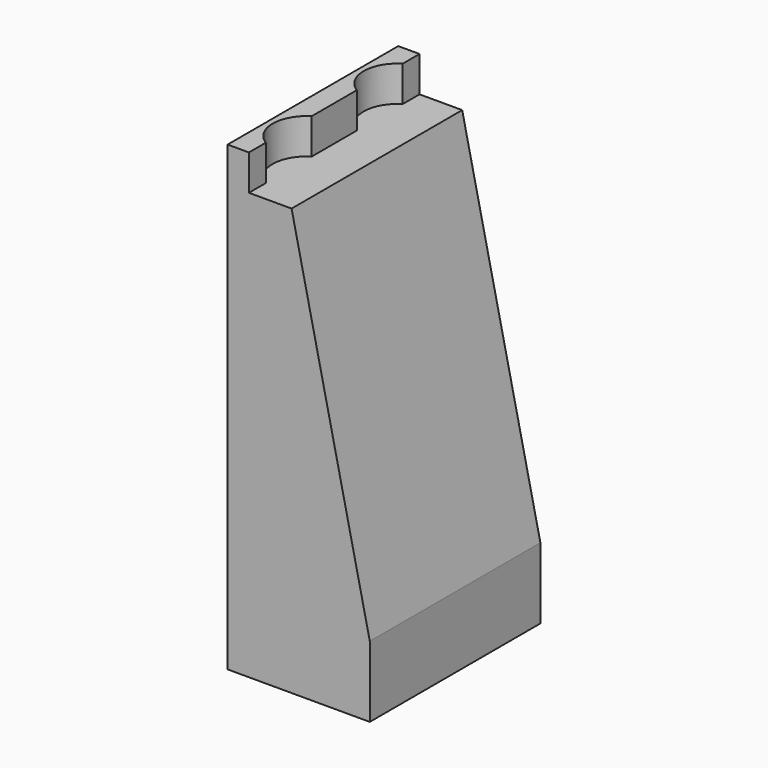
from build123d import *

# Parameters (mm, degrees)
F0_W      = 20
F0_H      = 70
F1_DEPTH  = 30
F2_W      = 30
F2_H      = 10
F3_DEPTH  = 10
F4_R      = 2.05
F5_DEPTH  = 10
F6_W      = 11
F6_H      = 30
F7_DEPTH  = 50
F9_DEPTH  = 5
F10_SIZE2 = 10.99999
F10_SIZE  = 49.99999
F11_W     = 30
F11_H     = 10
F12_DEPTH = 25


# Not quite as in the source:
# - a fillet or chamfer is up to 0.001 mm smaller than in the source, because OpenCascade refuses the exact size


with BuildPart() as f1:
    # F0 (on Front) → F1 (new body)
    with BuildSketch(Plane.XZ):
        with Locations((-10, 35)):
            Rectangle(F0_W, F0_H)
    extrude(amount=F1_DEPTH)

    # F2 (on face) → F3 (cut)
    with BuildSketch(Plane(origin=(-20, 0, 0), x_dir=(0, -1, 0), z_dir=(-1, 0, 0))):
        with Locations((15, 5)):
            Rectangle(F2_W, F2_H)
    extrude(amount=-F3_DEPTH, mode=Mode.SUBTRACT)

    # F4 (on face) → F5 (cut, through all)
    with BuildSketch(Plane(origin=(-10, 0, 0), x_dir=(0, -1, 0), z_dir=(-1, 0, 0))):
        with Locations((5, 5)):
            Circle(F4_R)
        with Locations((25, 5)):
            Circle(F4_R)
    extrude(amount=-F5_DEPTH, mode=Mode.SUBTRACT)

    # F6 (on face) → F7 (cut)
    with BuildSketch(Plane.XY.offset(70)):
        with Locations((-5.5, -15)):
            Rectangle(F6_W, F6_H)
    extrude(amount=-F7_DEPTH, mode=Mode.SUBTRACT)

    # F8 (on face) → F9 (join)
    with BuildSketch(Plane.XY.offset(70)):
        with BuildLine():
            ThreePointArc((-17, -11.0388736054), (-19.25, -7), (-17, -2.9611263946))
            Line((-17, -2.9611263946), (-17, 0))
            Line((-17, 0), (-20, 0))
            Line((-20, 0), (-20, -30))
            Line((-20, -30), (-17, -30))
            Line((-17, -30), (-17, -27.0388736054))
            ThreePointArc((-17, -27.0388736054), (-19.25, -23), (-17, -18.9611263946))
            Line((-17, -18.9611263946), (-17, -11.0388736054))
        make_face()
    extrude(amount=F9_DEPTH)

    # F10 (size 50 and 11 in the source; OpenCascade refuses exactly that, so slightly less here)
    f10_edges = [f1.edges().sort_by_distance(p)[0] for p in [
        (-11, -15, 20),
    ]]
    f10_side = f1.faces().sort_by_distance((-11, -15, 45))[0]
    chamfer(f10_edges, length=F10_SIZE, length2=F10_SIZE2, reference=f10_side)

    # F11 (on face) → F12 (cut)
    with BuildSketch(Plane(origin=(-10, 0, 0), x_dir=(0, -1, 0), z_dir=(-1, 0, 0))):
        with Locations((15, 5)):
            Rectangle(F11_W, F11_H)
    extrude(amount=-F12_DEPTH, mode=Mode.SUBTRACT)


solid = f1.part
